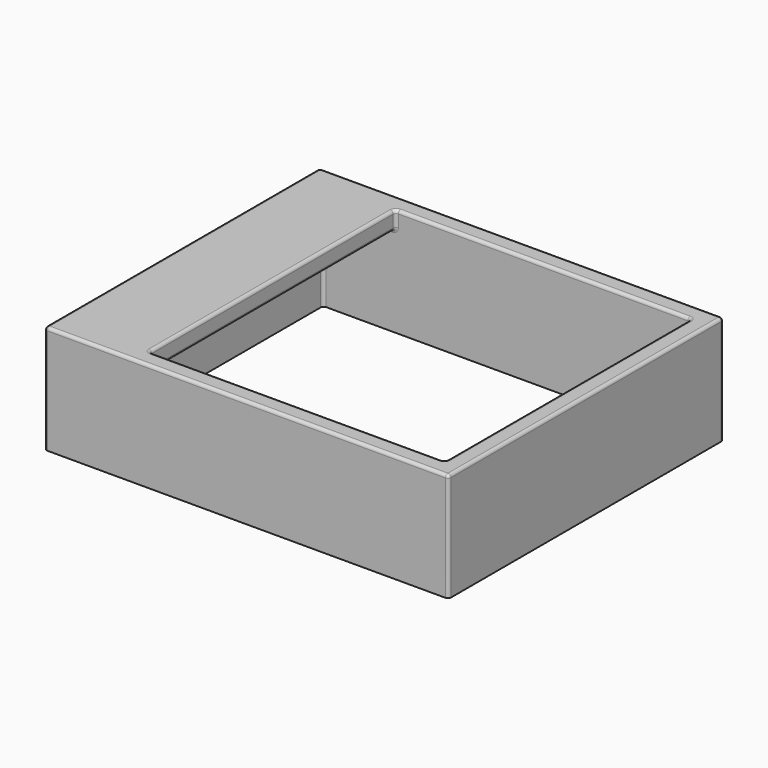
from build123d import *

# Parameters (mm, degrees)
F1_DEPTH = 15
F3_DEPTH = 3
F4_F1_R  = 0.5
F4_F2_R  = 0.5
F4_F3_R  = 0.5
F4_F4_R  = 0.5


with BuildPart() as f1:
    # F0 (on Top) → F1 (new body)
    with BuildSketch(Plane.XY):
        with BuildLine():
            Line((35.5372718227, 19.9606023237), (-30.4627281773, 19.9606023237))
            ThreePointArc((-30.4627281773, 19.9606023237), (-30.8162815679, 19.8141557143), (-30.9627281773, 19.4606023237))
            Line((-30.9627281773, 19.4606023237), (-30.9627281773, -36.5393976763))
            ThreePointArc((-30.9627281773, -36.5393976763), (-30.8162815679, -36.8929510669), (-30.4627281773, -37.0393976763))
            Line((-30.4627281773, -37.0393976763), (35.5372718227, -37.0393976763))
            ThreePointArc((35.5372718227, -37.0393976763), (35.8908252133, -36.8929510669), (36.0372718227, -36.5393976763))
            Line((36.0372718227, -36.5393976763), (36.0372718227, 19.4606023237))
            ThreePointArc((36.0372718227, 19.4606023237), (35.8908252133, 19.8141557143), (35.5372718227, 19.9606023237))
        make_face()
        with BuildLine():
            ThreePointArc((-27.9627281773, 16.4606023237), (-27.8162815679, 16.8141557143), (-27.4627281773, 16.9606023237))
            Line((-27.4627281773, 16.9606023237), (32.5372718227, 16.9606023237))
            ThreePointArc((32.5372718227, 16.9606023237), (32.8908252133, 16.8141557143), (33.0372718227, 16.4606023237))
            Line((33.0372718227, 16.4606023237), (33.0372718227, -33.5393976763))
            ThreePointArc((33.0372718227, -33.5393976763), (32.8908252133, -33.8929510669), (32.5372718227, -34.0393976763))
            Line((32.5372718227, -34.0393976763), (-27.4627281773, -34.0393976763))
            ThreePointArc((-27.4627281773, -34.0393976763), (-27.8162815679, -33.8929510669), (-27.9627281773, -33.5393976763))
            Line((-27.9627281773, -33.5393976763), (-27.9627281773, 16.4606023237))
        make_face(mode=Mode.SUBTRACT)
    extrude(amount=F1_DEPTH)

    # F2 (on face) → F3 (join)
    with BuildSketch(Plane.XY.offset(15)):
        with BuildLine():
            Line((-15.9627281773, -34.0393976763), (-15.9627281773, 16.9606023237))
            Line((-15.9627281773, 16.9606023237), (-27.4627281773, 16.9606023237))
            ThreePointArc((-27.4627281773, 16.9606023237), (-27.8162815679, 16.8141557143), (-27.9627281773, 16.4606023237))
            Line((-27.9627281773, 16.4606023237), (-27.9627281773, -33.5393976763))
            ThreePointArc((-27.9627281773, -33.5393976763), (-27.8162815679, -33.8929510669), (-27.4627281773, -34.0393976763))
            Line((-27.4627281773, -34.0393976763), (-15.9627281773, -34.0393976763))
        make_face()
        with BuildLine():
            ThreePointArc((-30.4627281773, 19.9606023237), (-30.8162815679, 19.8141557143), (-30.9627281773, 19.4606023237))
            Line((-30.9627281773, 19.4606023237), (-30.9627281773, -36.5393976763))
            ThreePointArc((-30.9627281773, -36.5393976763), (-30.8162815679, -36.8929510669), (-30.4627281773, -37.0393976763))
            Line((-30.4627281773, -37.0393976763), (-15.9627281773, -37.0393976763))
            Line((-15.9627281773, -37.0393976763), (-15.9627281773, -34.0393976763))
            Line((-15.9627281773, -34.0393976763), (-27.4627281773, -34.0393976763))
            ThreePointArc((-27.4627281773, -34.0393976763), (-27.8162815679, -33.8929510669), (-27.9627281773, -33.5393976763))
            Line((-27.9627281773, -33.5393976763), (-27.9627281773, 16.4606023237))
            ThreePointArc((-27.9627281773, 16.4606023237), (-27.8162815679, 16.8141557143), (-27.4627281773, 16.9606023237))
            Line((-27.4627281773, 16.9606023237), (-15.9627281773, 16.9606023237))
            Line((-15.9627281773, 16.9606023237), (-15.9627281773, 19.9606023237))
            Line((-15.9627281773, 19.9606023237), (-30.4627281773, 19.9606023237))
        make_face()
        with BuildLine():
            Line((35.5372718227, 19.9606023237), (-15.9627281773, 19.9606023237))
            Line((-15.9627281773, 19.9606023237), (-15.9627281773, 16.9606023237))
            Line((-15.9627281773, 16.9606023237), (32.5372718227, 16.9606023237))
            ThreePointArc((32.5372718227, 16.9606023237), (32.8908252133, 16.8141557143), (33.0372718227, 16.4606023237))
            Line((33.0372718227, 16.4606023237), (33.0372718227, -33.5393976763))
            ThreePointArc((33.0372718227, -33.5393976763), (32.8908252133, -33.8929510669), (32.5372718227, -34.0393976763))
            Line((32.5372718227, -34.0393976763), (-15.9627281773, -34.0393976763))
            Line((-15.9627281773, -34.0393976763), (-15.9627281773, -37.0393976763))
            Line((-15.9627281773, -37.0393976763), (35.5372718227, -37.0393976763))
            ThreePointArc((35.5372718227, -37.0393976763), (35.8908252133, -36.8929510669), (36.0372718227, -36.5393976763))
            Line((36.0372718227, -36.5393976763), (36.0372718227, 19.4606023237))
            ThreePointArc((36.0372718227, 19.4606023237), (35.8908252133, 19.8141557143), (35.5372718227, 19.9606023237))
        make_face()
    extrude(amount=F3_DEPTH)

    # F4: fillet of radius 0.5 on 7 edges, made by hand

    # F4_f1
    f4_f1_edges = [f1.edges().sort_by_distance(p)[0] for p in [
        (2.5372718227, 19.9606023237, 18),
        (36.0372718227, -8.5393976763, 18),
        (35.8908252133, -36.8929510669, 18),
        (2.5372718227, -37.0393976763, 18),
        (-30.8162815679, -36.8929510669, 18),
        (-30.9627281773, -8.5393976763, 18),
        (-30.8162815679, 19.8141557143, 18),
        (35.8908252133, 19.8141557143, 18),
    ]]
    fillet(f4_f1_edges, radius=F4_F1_R)

    # F4_f2
    f4_f2_edges = [f1.edges().sort_by_distance(p)[0] for p in [
        (-15.9627281773, -8.5393976763, 15),
    ]]
    fillet(f4_f2_edges, radius=F4_F2_R)

    # F4_f3
    f4_f3_edges = [f1.edges().sort_by_distance(p)[0] for p in [
        (-15.9627281773, -34.0393976763, 16.75),
    ]]
    fillet(f4_f3_edges, radius=F4_F3_R)

    # F4_f4
    f4_f4_edges = [f1.edges().sort_by_distance(p)[0] for p in [
        (-15.9627281773, -8.5393976763, 18),
    ]]
    fillet(f4_f4_edges, radius=F4_F4_R)


solid = f1.part
